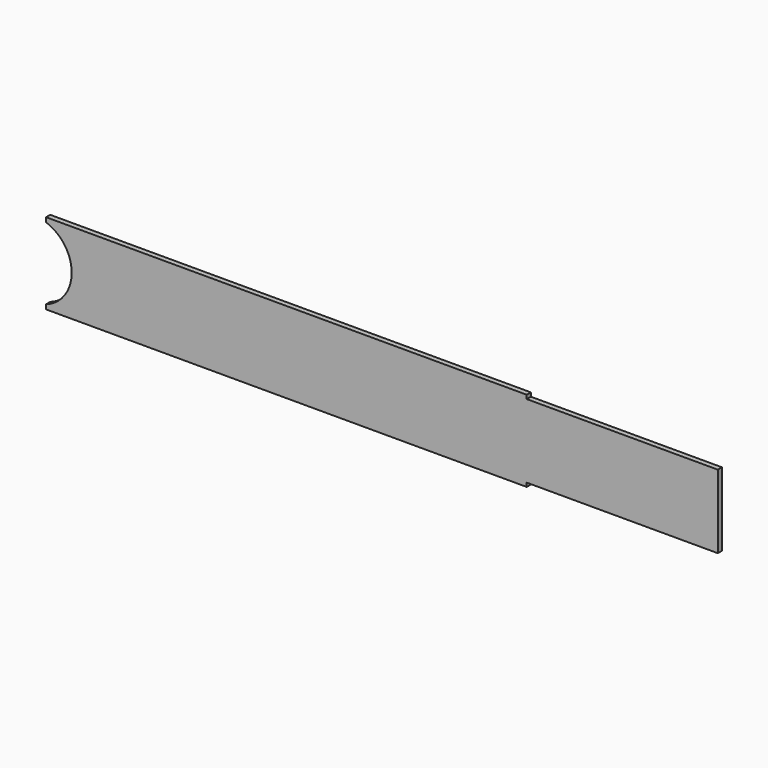
from build123d import *

# Parameters (mm, degrees)
F1_DEPTH = 3.429


# Not quite as in the source:
# - ends of sketch curves that miss each other by under 0.0002 mm in the source are joined


with BuildPart() as f1:
    # F0 (on Front) → F1 (new body)
    with BuildSketch(Plane.XZ):
        with BuildLine():
            Line((758.6498162, 426.3902572), (758.6498162, 428.9302572))
            Line((758.6498162, 428.9302572), (439.1178162, 428.9302572))
            Line((439.1178162, 428.9302572), (439.1178162, 425.9198746))
            ThreePointArc((439.1178162, 425.9198746), (456.1358162, 401.9427572), (439.117815662, 377.9656413389))
            Line((439.117815662, 377.9656413389), (439.1178162, 374.9552572))
            Line((439.1178162, 374.9552572), (758.6498162, 374.9552572))
            Line((758.6498162, 374.9552572), (758.6498162, 377.4952572))
            Line((758.6498162, 377.4952572), (885.6498162, 377.4952572))
            Line((885.6498162, 377.4952572), (885.6498162, 426.3902572))
            Line((885.6498162, 426.3902572), (758.6498162, 426.3902572))
        make_face()
    extrude(amount=F1_DEPTH)


solid = f1.part
